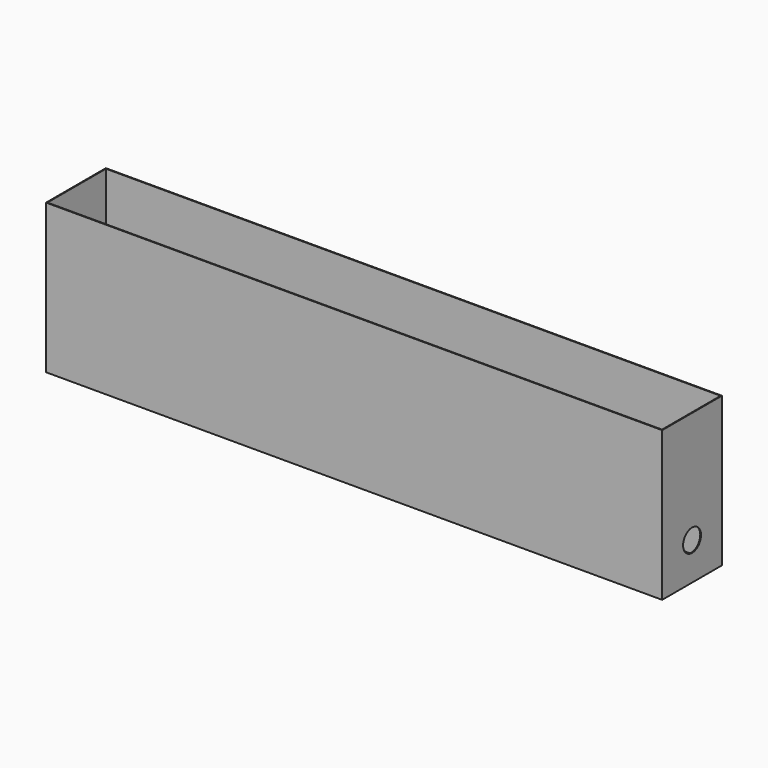
from build123d import *

# Parameters (mm, degrees)
F0_W     = 825
F0_H     = 100
F1_DEPTH = 200
F2_T     = -1
F5_D     = 20
F8_D     = 30


# Not quite as in the source:
# - the program builds the solid bodies; features that only make, move or delete a surface that nothing else refers to are left out


with BuildPart() as f1:
    # F0 (on Top) → F1 (new body)
    with BuildSketch(Plane.XY):
        Rectangle(F0_W, F0_H)
    extrude(amount=F1_DEPTH)

    # F2
    f2_openings = [f1.faces().sort_by_distance(p)[0] for p in [
        (0, 0, 200),
    ]]
    offset(amount=F2_T, openings=f2_openings)

    # F5 (through all)
    with Locations(Plane.XY.offset(1)):
        with Locations((399.5, 37), (399.5, -37), (-399.5, 37), (-399.5, -37)):
            Hole(F5_D / 2)

    # F8 (through all)
    with Locations(Plane(origin=(-412.5, 0, 0), x_dir=(0, -1, 0), z_dir=(-1, 0, 0))):
        with Locations((0, 50)):
            Hole(F8_D / 2)


solid = f1.part
